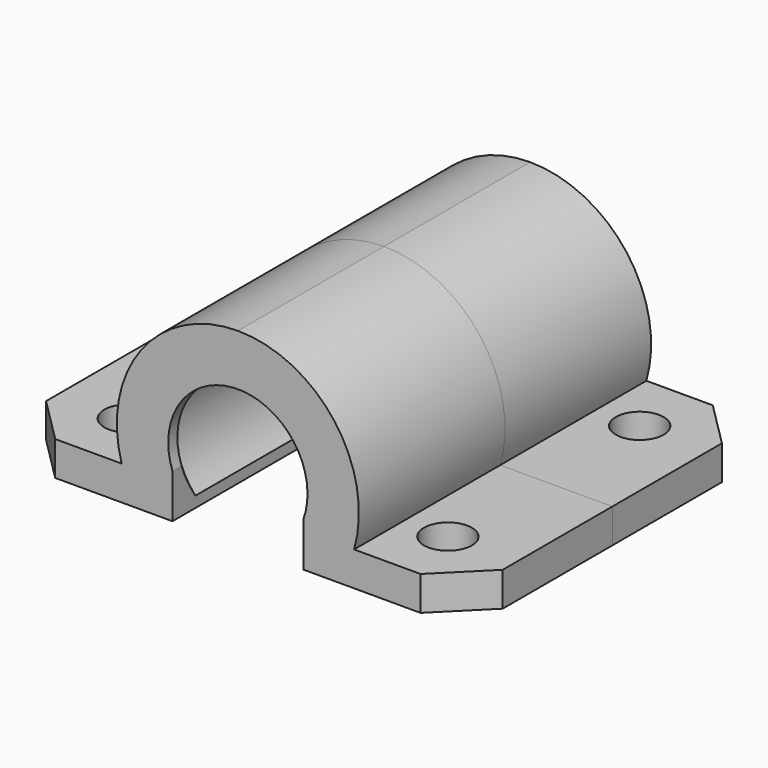
from build123d import *

# Parameters (mm, degrees)
F1_DEPTH = 16
F2_R     = 2.1
F3_DEPTH = 3
F4_SIZE  = 4
F6_DEPTH = 2.5
F7_SIZE  = 1.49999


# Not quite as in the source:
# - a fillet or chamfer is up to 0.001 mm smaller than in the source, because OpenCascade refuses the exact size


with BuildPart() as f1:
    # F0 (on Front) → F1 (new body)
    with BuildSketch(Plane.XZ):
        with BuildLine():
            ThreePointArc((-5.7283718128, -4.9945726919), (-6.9180471398, 3.1465256666), (0, 7.6))
            Line((0, 7.6), (0, 10.6))
            ThreePointArc((0, 10.6), (-8.4743731332, 6.367495583), (-10.1812327348, -2.95))
            Line((-10.1812327348, -2.95), (-20, -2.95))
            Line((-20, -2.95), (-20, -5.95))
            Line((-20, -5.95), (-5.7283718128, -5.95))
            Line((-5.7283718128, -5.95), (-5.7283718128, -4.9945726919))
        make_face()
        with BuildLine():
            Line((0, 10.6), (0, 7.6))
            ThreePointArc((0, 7.6), (6.9180471398, 3.1465256666), (5.7283718128, -4.9945726919))
            Line((5.7283718128, -4.9945726919), (5.7283718128, -5.95))
            Line((5.7283718128, -5.95), (20, -5.95))
            Line((20, -5.95), (20, -2.95))
            Line((20, -2.95), (10.1812327348, -2.95))
            ThreePointArc((10.1812327348, -2.95), (8.4743731332, 6.367495583), (0, 10.6))
        make_face()
    extrude(amount=F1_DEPTH)

    # F2 (on face) → F3 (cut, through all)
    with BuildSketch(Plane.XY.offset(-2.95)):
        with Locations((-14, -10.5)):
            Circle(F2_R)
        with Locations((14, -10.5)):
            Circle(F2_R)
    extrude(amount=-F3_DEPTH, mode=Mode.SUBTRACT)

    # F4
    f4_edges = [f1.edges().sort_by_distance(p)[0] for p in [
        (-20, -16, -4.45),
        (20, -16, -4.45),
    ]]
    chamfer(f4_edges, length=F4_SIZE)

    # F5 (on face) → F6 (join)
    with BuildSketch(Plane.XZ.offset(16)):
        with BuildLine():
            Line((5.7283718128, -2.0966059178), (5.7283718128, -4.9945726919))
            ThreePointArc((5.7283718128, -4.9945726919), (0, 7.6), (-5.7283718128, -4.9945726919))
            Line((-5.7283718128, -4.9945726919), (-5.7283718128, -2.0966059178))
            ThreePointArc((-5.7283718128, -2.0966059178), (0, 6.1), (5.7283718128, -2.0966059178))
        make_face()
    extrude(amount=-F6_DEPTH)

    # F7 (size 1.5 in the source; OpenCascade refuses exactly that, so slightly less here)
    f7_edges = [f1.edges().sort_by_distance(p)[0] for p in [
        (0, -13.5, 6.1),
    ]]
    chamfer(f7_edges, length=F7_SIZE)

    # F8: F1 across plane


with BuildPart() as f1_1:
    add(f1.part)
    add(f1.part.mirror(Plane.XZ))


solid = f1_1.part
